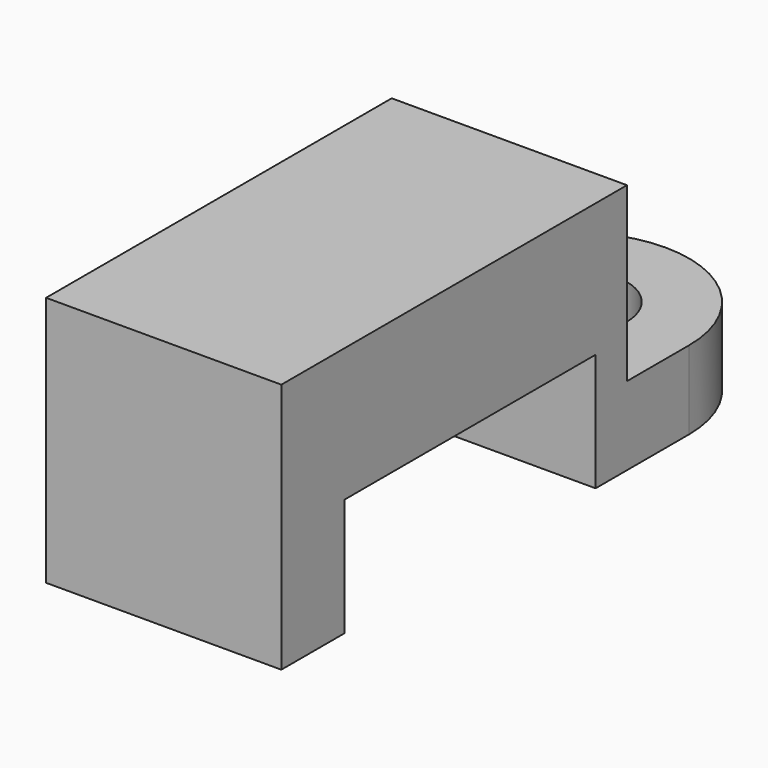
from build123d import *

# Parameters (mm, degrees)
F0_W     = 6
F0_H     = 16
F0_R     = 1.4
F1_DEPTH = 6.4
F2_R     = 2.99999
F3_W     = 1.9810468791
F3_H     = 4.4
F3_W_2   = 8
F3_H_2   = 3
F4_DEPTH = 8


# Not quite as in the source:
# - a fillet or chamfer is up to 0.001 mm smaller than in the source, because OpenCascade refuses the exact size


with BuildPart() as f1:
    # F0 (on Top) → F1 (new body)
    with BuildSketch(Plane.XY):
        Rectangle(F0_W, F0_H)
        with Locations((0, 5)):
            Circle(F0_R, mode=Mode.SUBTRACT)
    extrude(amount=F1_DEPTH)

    # F2 (radius 3 in the source; OpenCascade refuses exactly that, so slightly less here)
    f2_edges = [f1.edges().sort_by_distance(p)[0] for p in [
        (3, 8, 3.2),
        (-3, 8, 3.2),
    ]]
    fillet(f2_edges, radius=F2_R)

    # F3 (on face) → F4 (cut)
    with BuildSketch(Plane.YZ.offset(3)):
        Polygon((5.00001, 6.4), (5.00001, 2), (8.0189631209, 2), (8.0189631209, 7), (3.0189631209, 7), (3.0189631209, 6.4), align=None)
        with Locations((4.0094865604, 4.2)):
            Rectangle(F3_W, F3_H)
        with Locations((-1.9810368791, 1.5)):
            Rectangle(F3_W_2, F3_H_2)
    extrude(amount=-F4_DEPTH, mode=Mode.SUBTRACT)


solid = f1.part
